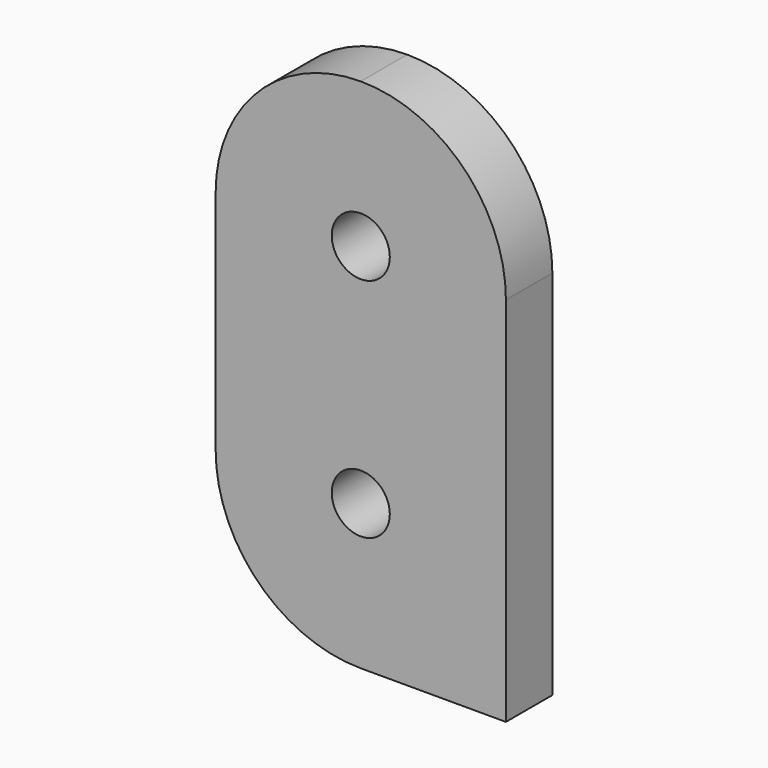
from build123d import *

# Parameters (mm, degrees)
F0_W     = 10
F0_H     = 17.8
F0_R     = 1
F1_DEPTH = 2
F2_R     = 4.99999


# Not quite as in the source:
# - a fillet or chamfer is up to 0.001 mm smaller than in the source, because OpenCascade refuses the exact size


with BuildPart() as f1:
    # F0 (on Front) → F1 (new body)
    with BuildSketch(Plane.XZ):
        with Locations((5, 8.9)):
            Rectangle(F0_W, F0_H)
        with Locations((5, 5)):
            Circle(F0_R, mode=Mode.SUBTRACT)
        with Locations((5, 12.8)):
            Circle(F0_R, mode=Mode.SUBTRACT)
    extrude(amount=F1_DEPTH)

    # F2 (radius 5 in the source; OpenCascade refuses exactly that, so slightly less here)
    f2_edges = [f1.edges().sort_by_distance(p)[0] for p in [
        (0, -1, 17.8),
        (10, -1, 17.8),
        (0, -1, 0),
    ]]
    fillet(f2_edges, radius=F2_R)


solid = f1.part
